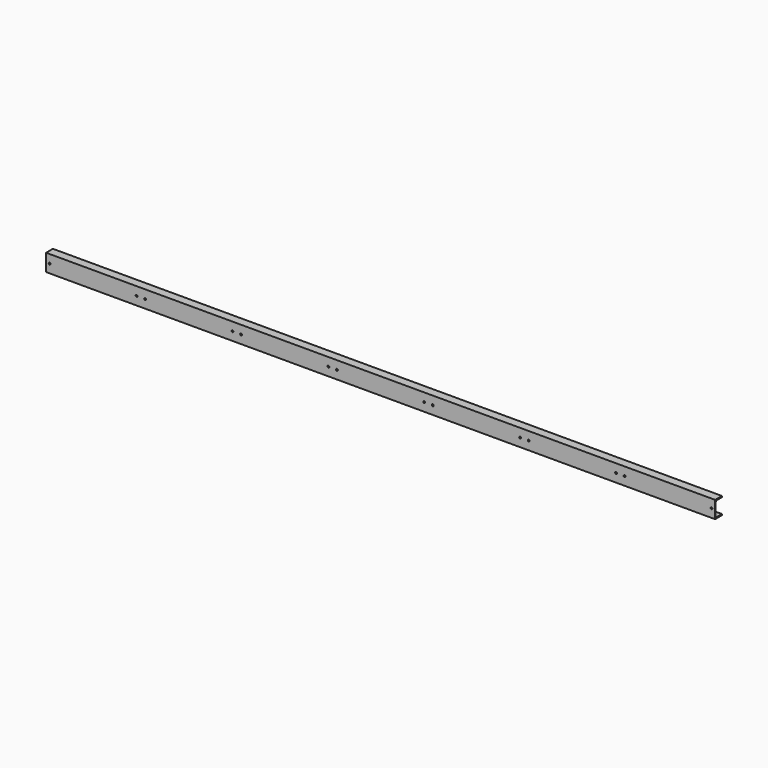
from build123d import *

# Parameters (mm, degrees)
F3_DEPTH = 4710
F4_R     = 6.5
F5_DEPTH = 8
F6_R     = 6.5
F7_DEPTH = 60.001


with BuildPart() as f3:
    # F2 (on Right) → F3 (new body)
    with BuildSketch(Plane.YZ):
        with BuildLine():
            Line((-60, 0), (0, 0))
            Line((0, 0), (0, 8))
            Line((0, 8), (-43, 8))
            ThreePointArc((-43, 8), (-51.4852813742, 11.5147186258), (-55, 20))
            Line((-55, 20), (-55, 100))
            ThreePointArc((-55, 100), (-51.4852813742, 108.4852813742), (-43, 112))
            Line((-43, 112), (0, 112))
            Line((0, 112), (0, 120))
            Line((0, 120), (-60, 120))
            Line((-60, 120), (-60, 0))
        make_face()
    extrude(amount=-F3_DEPTH)

    # F4 (on face) → F5 (cut, through all)
    with BuildSketch(Plane.XY.offset(8)):
        with Locations((-85, -20)):
            Circle(F4_R)
        with Locations((-4625, -20)):
            Circle(F4_R)
    extrude(amount=-F5_DEPTH, mode=Mode.SUBTRACT)

    # F6 (on face) → F7 (cut, through all)
    with BuildSketch(Plane.XZ.offset(60)):
        with Locations((-2047.5, 60)):
            Circle(F6_R)
        with Locations((-1987.5, 60)):
            Circle(F6_R)
        with Locations((-1372.5, 60)):
            Circle(F6_R)
        with Locations((-1312.5, 60)):
            Circle(F6_R)
        with Locations((-697.5, 60)):
            Circle(F6_R)
        with Locations((-637.5, 60)):
            Circle(F6_R)
        with Locations((-25, 60)):
            Circle(F6_R)
        with Locations((-2662.5, 60)):
            Circle(F6_R)
        with Locations((-2722.5, 60)):
            Circle(F6_R)
        with Locations((-3337.5, 60)):
            Circle(F6_R)
        with Locations((-3397.5, 60)):
            Circle(F6_R)
        with Locations((-4012.5, 60)):
            Circle(F6_R)
        with Locations((-4072.5, 60)):
            Circle(F6_R)
        with Locations((-4685, 60)):
            Circle(F6_R)
    extrude(amount=-F7_DEPTH, mode=Mode.SUBTRACT)


solid = f3.part
